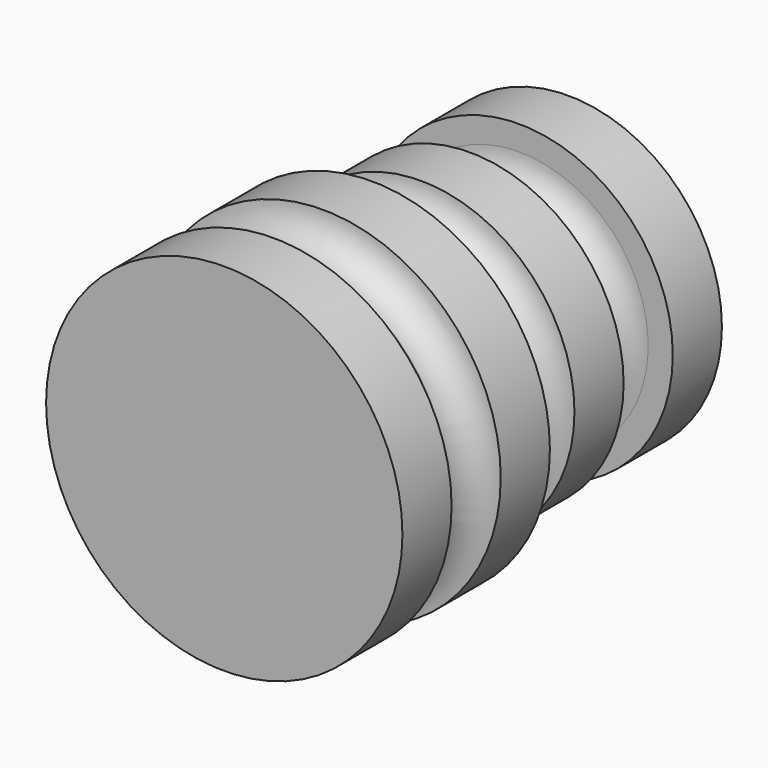
from build123d import *

# Parameters (mm, degrees)
F0_W   = 12
F0_H   = 5
F0_W_2 = 10
F0_W_3 = 8
F2_R   = 2.49999


# Not quite as in the source:
# - a fillet or chamfer is up to 0.001 mm smaller than in the source, because OpenCascade refuses the exact size


with BuildPart() as f1:
    # F0 (on Top) → F1 (revolve)
    with BuildSketch(Plane.XY):
        Polygon((-11.1182456035, -9.2245248563), (-11.1182456035, -14.2245248563), (3.3817543965, -14.2245248563), (3.3817543965, -9.2245248563), (-8.6182456035, -9.2245248563), align=None)
        with Locations((-2.6182456035, -6.7245248563)):
            Rectangle(F0_W, F0_H)
        Polygon((-8.6182456035, -4.2245248563), (3.3817543965, -4.2245248563), (3.3817543965, 0.7754751437), (-6.6182456035, 0.7754751437), (-11.1182456035, 0.7754751437), (-11.1182456035, -4.2245248563), align=None)
        with Locations((-1.6182456035, 3.2754751437)):
            Rectangle(F0_W_2, F0_H)
        Polygon((-6.6182456035, 5.7754751437), (3.3817543965, 5.7754751437), (3.3817543965, 10.7754751437), (-4.6182456035, 10.7754751437), (-9.1182456035, 10.7754751437), (-9.1182456035, 5.7754751437), align=None)
        with Locations((-0.6182456035, 13.2754751437)):
            Rectangle(F0_W_3, F0_H)
        Polygon((-4.6182456035, 15.7754751437), (3.3817543965, 15.7754751437), (3.3817543965, 20.7754751437), (-9.1182456035, 20.7754751437), (-9.1182456035, 15.7754751437), align=None)
    revolve(axis=Axis((3.3817543965, 3.2754751437, 0), (0, 1, 0)))

    # F2 (radius 2.5 in the source; OpenCascade refuses exactly that, so slightly less here)
    f2_edges = [f1.edges().sort_by_distance(p)[0] for p in [
        (11.381754, 15.775475, 0),
        (11.381754, 10.775475, 0),
        (13.381754, 5.775475, 0),
        (13.381754, 0.775475, 0),
        (15.381754, -4.224525, 0),
        (15.381754, -9.224525, 0),
    ]]
    fillet(f2_edges, radius=F2_R)


solid = f1.part
